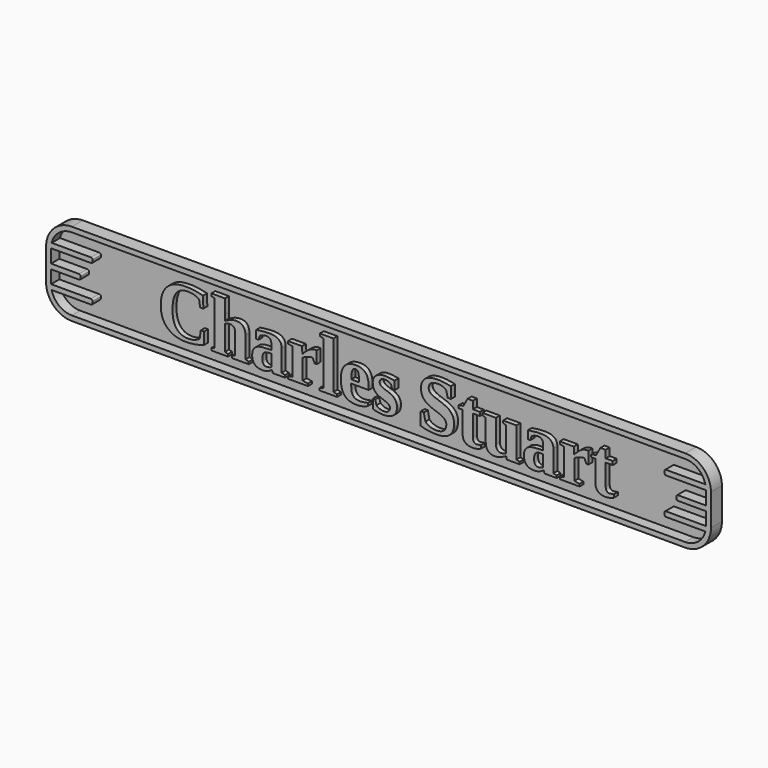
from build123d import *

# Parameters (mm, degrees)
F1_DEPTH     = 3.175
F3_DEPTH     = 1.016
F4_TEXT_SIZE = 22.1472957896
F5_DEPTH     = 1.524


# Not quite as in the source:
# - Text() gives the source's letters only with a copy of the font that has no kerning and outlines rounded to 1/6400 em; it was checked with that copy


with BuildPart() as f1:
    # F0 (on Front) → F1 (new body)
    with BuildSketch(Plane.XZ):
        with BuildLine():
            Line((93.726, -23.3766014767), (-93.726, -23.3766014767))
            ThreePointArc((-93.726, -23.3766014767), (-99.2937587951, -25.6828426817), (-101.6, -31.2506014767))
            Line((-101.6, -31.2506014767), (-101.6, -40.9026014767))
            ThreePointArc((-101.6, -40.9026014767), (-99.2937587951, -46.4703602718), (-93.726, -48.7766014767))
            Line((-93.726, -48.7766014767), (93.726, -48.7766014767))
            ThreePointArc((93.726, -48.7766014767), (99.2937587951, -46.4703602718), (101.6, -40.9026014767))
            Line((101.6, -40.9026014767), (101.6, -31.2506014767))
            ThreePointArc((101.6, -31.2506014767), (99.2937587951, -25.6828426817), (93.726, -23.3766014767))
        make_face()
        with BuildLine():
            ThreePointArc((-99.8904078386, -29.7266014767), (-97.6404028919, -26.2506064767), (-93.726, -24.9006014767))
            Line((-93.726, -24.9006014767), (93.726, -24.9006014767))
            ThreePointArc((93.726, -24.9006014767), (97.6404028919, -26.2506064767), (99.8904078386, -29.7266014767))
            Line((99.8904078386, -29.7266014767), (87.884, -29.7266014767))
            ThreePointArc((87.884, -29.7266014767), (87.5247897552, -29.8753912319), (87.376, -30.2346014767))
            Line((87.376, -30.2346014767), (87.376, -30.7426014767))
            ThreePointArc((87.376, -30.7426014767), (87.5247897552, -31.1018117216), (87.884, -31.2506014767))
            Line((87.884, -31.2506014767), (100.076, -31.2506014767))
            Line((100.076, -31.2506014767), (100.076, -35.3772840092))
            Line((100.076, -35.3772840092), (91.524383482, -35.3772840092))
            ThreePointArc((91.524383482, -35.3772840092), (91.1651732371, -35.5260737644), (91.016383482, -35.8852840092))
            Line((91.016383482, -35.8852840092), (91.016383482, -36.3932840092))
            ThreePointArc((91.016383482, -36.3932840092), (91.1651732371, -36.7524942541), (91.524383482, -36.9012840092))
            Line((91.524383482, -36.9012840092), (100.076, -36.9012840092))
            Line((100.076, -36.9012840092), (100.076, -40.9026014767))
            Line((100.076, -40.9026014767), (87.884, -40.9026014767))
            ThreePointArc((87.884, -40.9026014767), (87.5247897552, -41.0513912319), (87.376, -41.4106014767))
            Line((87.376, -41.4106014767), (87.376, -41.9137022955))
            ThreePointArc((87.376, -41.9137022955), (87.5247897552, -42.2729125404), (87.884, -42.4217022955))
            Line((87.884, -42.4217022955), (99.8916169766, -42.4217022955))
            ThreePointArc((99.8916169766, -42.4217022955), (97.6423892682, -45.9010407431), (93.726, -47.2526014767))
            Line((93.726, -47.2526014767), (-93.726, -47.2526014767))
            ThreePointArc((-93.726, -47.2526014767), (-97.6423892682, -45.9010407431), (-99.8916169766, -42.4217022955))
            Line((-99.8916169766, -42.4217022955), (-87.884, -42.4217022955))
            ThreePointArc((-87.884, -42.4217022955), (-87.5247897552, -42.2729125404), (-87.376, -41.9137022955))
            Line((-87.376, -41.9137022955), (-87.376, -41.4106014767))
            ThreePointArc((-87.376, -41.4106014767), (-87.5247897552, -41.0513912319), (-87.884, -40.9026014767))
            Line((-87.884, -40.9026014767), (-100.076, -40.9026014767))
            Line((-100.076, -40.9026014767), (-100.076, -36.9012840092))
            Line((-100.076, -36.9012840092), (-91.524383482, -36.9012840092))
            ThreePointArc((-91.524383482, -36.9012840092), (-91.1651732371, -36.7524942541), (-91.016383482, -36.3932840092))
            Line((-91.016383482, -36.3932840092), (-91.016383482, -35.8852840092))
            ThreePointArc((-91.016383482, -35.8852840092), (-91.1651732371, -35.5260737644), (-91.524383482, -35.3772840092))
            Line((-91.524383482, -35.3772840092), (-100.076, -35.3772840092))
            Line((-100.076, -35.3772840092), (-100.076, -31.2506014767))
            Line((-100.076, -31.2506014767), (-87.884, -31.2506014767))
            ThreePointArc((-87.884, -31.2506014767), (-87.5247897552, -31.1018117216), (-87.376, -30.7426014767))
            Line((-87.376, -30.7426014767), (-87.376, -30.2346014767))
            ThreePointArc((-87.376, -30.2346014767), (-87.5247897552, -29.8753912319), (-87.884, -29.7266014767))
            Line((-87.884, -29.7266014767), (-99.8904078386, -29.7266014767))
        make_face(mode=Mode.SUBTRACT)
    extrude(amount=F1_DEPTH)

    # F2 (on face) → F3 (join)
    with BuildSketch(Plane(origin=(0, 0, 0), x_dir=(-1, 0, 0), z_dir=(0, 1, 0))):
        with BuildLine():
            ThreePointArc((101.6, -31.2506014767), (99.2937587951, -25.6828426817), (93.726, -23.3766014767))
            Line((93.726, -23.3766014767), (-93.726, -23.3766014767))
            ThreePointArc((-93.726, -23.3766014767), (-99.2937587951, -25.6828426817), (-101.6, -31.2506014767))
            Line((-101.6, -31.2506014767), (-101.6, -40.9026014767))
            ThreePointArc((-101.6, -40.9026014767), (-99.2937587951, -46.4703602718), (-93.726, -48.7766014767))
            Line((-93.726, -48.7766014767), (93.726, -48.7766014767))
            ThreePointArc((93.726, -48.7766014767), (99.2937587951, -46.4703602718), (101.6, -40.9026014767))
            Line((101.6, -40.9026014767), (101.6, -31.2506014767))
        make_face()
    extrude(amount=F3_DEPTH)

    # F4 (on face) → F5 (join)
    with BuildSketch(Plane.XZ):
        with Locations((-68.9596710727, -43.9215768129)):
            Text('Charles Stuart', F4_TEXT_SIZE, font='Tinos', font_style=FontStyle.BOLD, text_align=(TextAlign.LEFT, TextAlign.BOTTOM))
    extrude(amount=F5_DEPTH)


solid = f1.part
